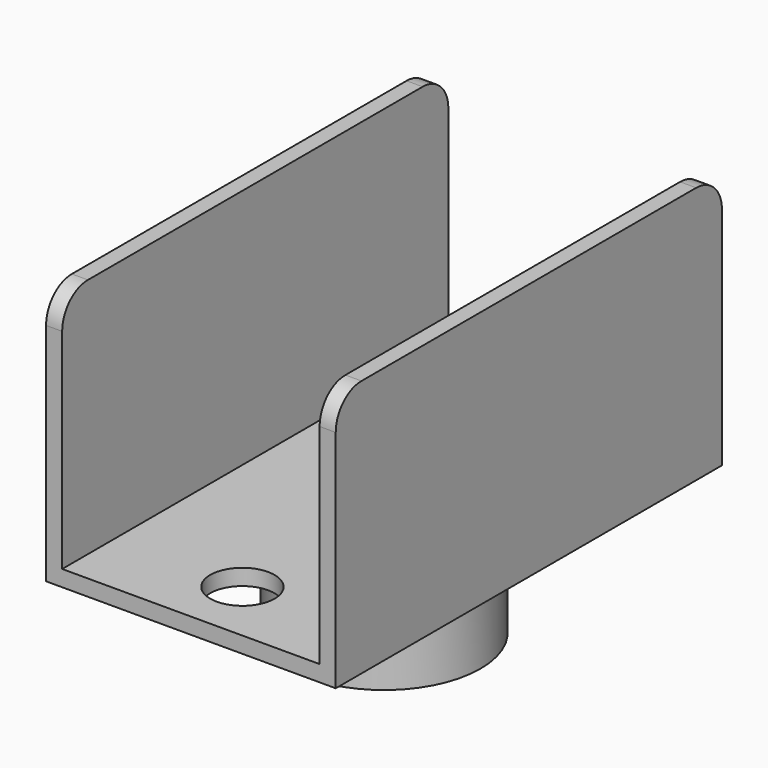
from build123d import *

# Parameters (mm, degrees)
F1_DEPTH = 30
F2_R     = 2.5
F3_DEPTH = 3
F4_R     = 6
F4_R_2   = 2.5
F5_DEPTH = 4
F6_R     = 2
F7_D     = 4
F7_DEPTH = 15
F7_TIP   = 1.2017212381


with BuildPart() as f1:
    # F0 (on Front) → F1 (new body)
    with BuildSketch(Plane.XZ):
        Polygon((0, 1), (0, 0), (18, 0), (18, 1), (18, 16), (17, 16), (17, 1), (1, 1), (1, 16), (0, 16), align=None)
    extrude(amount=-F1_DEPTH)

    # F2 (on face) → F3 (join)
    with BuildSketch(Plane.XY.offset(1)):
        with Locations((9, 15)):
            Circle(F2_R)
    extrude(amount=-F3_DEPTH)

    # F4 (on face) → F5 (join)
    with BuildSketch(Plane(origin=(0, 0, -2), x_dir=(1, 0, 0), z_dir=(0, 0, -1))):
        with Locations((9, -15)):
            Circle(F4_R)
        with Locations((9, -15)):
            Circle(F4_R_2, mode=Mode.SUBTRACT)
        with Locations((9, -15)):
            Circle(F4_R_2)
    extrude(amount=F5_DEPTH)

    # F6
    f6_edges = [f1.edges().sort_by_distance(p)[0] for p in [
        (17.5, 0, 16),
        (17.5, 30, 16),
        (0.5, 30, 16),
        (0.5, 0, 16),
    ]]
    fillet(f6_edges, radius=F6_R)

    # F7
    with Locations(Plane.XY.offset(1)):
        with Locations((9, 4), (9, 26)):
            Hole(F7_D / 2, depth=F7_DEPTH)
            with Locations((0, 0, -(F7_DEPTH + F7_TIP / 2))):  # 118° drill point
                Cone(0, F7_D / 2, F7_TIP, mode=Mode.SUBTRACT)


solid = f1.part
